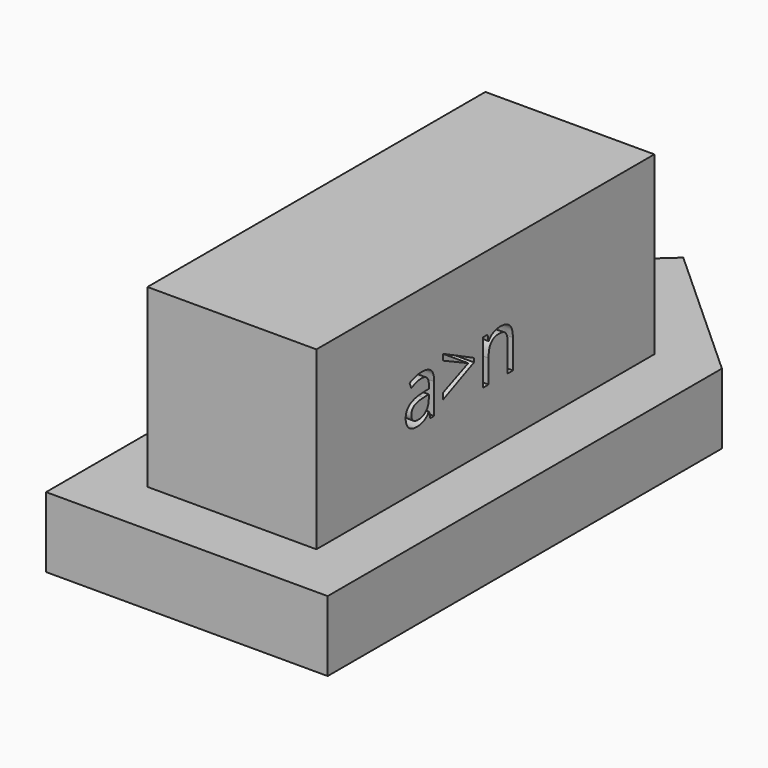
from build123d import *

# Parameters (mm, degrees)
F1_DEPTH     = 10
F2_W         = 24
F2_H         = 60
F3_DEPTH     = 25
F6_TEXT_SIZE = 11.7865209985
F7_DEPTH     = 5


# Not quite as in the source:
# - the program builds the solid bodies; features that only make, move or delete a surface that nothing else refers to are left out
# - Text() gives the source's letters only with a copy of the font that has no kerning and outlines rounded to 1/6400 em; it was checked with that copy


with BuildPart() as f1:
    # F0 (on Top) → F1 (new body)
    with BuildSketch(Plane.XY):
        Polygon((10.025319475, 37.0503156017), (-9.974680525, 55.1886727489), (-29.974680525, 37.0503156017), (-29.974680525, -32.9496843983), (10.025319475, -32.9496843983), align=None)
    extrude(amount=F1_DEPTH)

    # F2 (on face) → F3 (join)
    with BuildSketch(Plane.XY.offset(10)):
        with Locations((-9.974680525, 5.0503156017)):
            Rectangle(F2_W, F2_H)
    extrude(amount=F3_DEPTH)

    # F6 (on face) → F7 (cut)
    with BuildSketch(Plane.YZ.offset(2.025319475)):
        with Locations((-9.6436650492, 18.1759819388)):
            Text('a>n', F6_TEXT_SIZE, font='Open Sans', text_align=(TextAlign.LEFT, TextAlign.BOTTOM))
    extrude(amount=-F7_DEPTH, mode=Mode.SUBTRACT)


solid = f1.part
